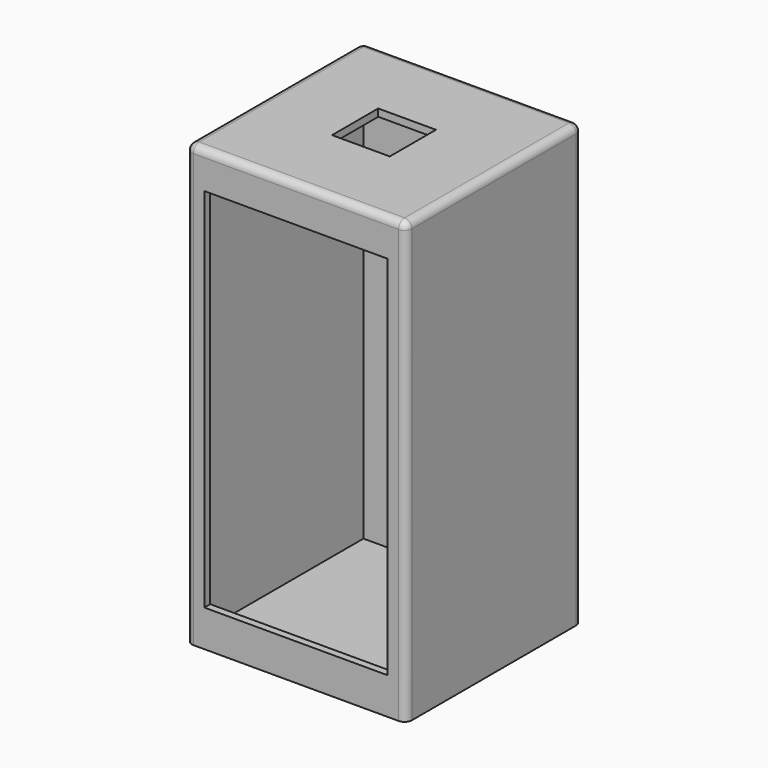
from build123d import *

# Parameters (mm, degrees)
F0_W     = 152.4
F0_H     = 304.8
F1_DEPTH = 76.2
F2_R     = 5.08
F3_T     = 5.08
F4_W     = 127
F4_H     = 254
F5_DEPTH = 25.4
F6_W     = 40
F6_H     = 40
F7_DEPTH = 5.08


# Not quite as in the source:
# - a shell that OpenCascade refuses in one call is made with other operations: the cavity is built on its own and cut out


with BuildPart() as f1:
    # F0 (on Front) → F1 (new body, symmetric)
    with BuildSketch(Plane.XZ):
        Rectangle(F0_W, F0_H)
    extrude(amount=F1_DEPTH, both=True)

    # F2
    f2_edges = [f1.edges().sort_by_distance(p)[0] for p in [
        (0, -76.2, 152.4),
        (76.2, 0, 152.4),
        (76.2, -76.2, 0),
        (76.2, 76.2, 0),
        (0, 76.2, 152.4),
        (-76.2, 0, 152.4),
        (-76.2, -76.2, 0),
        (-76.2, 76.2, 0),
    ]]
    fillet(f2_edges, radius=F2_R)

    # F3: shell of thickness 5.08, made by hand


with BuildPart() as f3_core1:
    # F3_t2: copy of F1
    add(f1.part)

    # the walls: a layer under each face that stays
    f3_faces = [f3_core1.faces().sort_by_distance(p)[0] for p in [
        (0, 0, -152.4),
        (0, 76.2, -2.54),
        (-76.2, 0, -2.54),
        (76.2, 0, -2.54),
        (0, -76.2, -2.54),
        (0, 0, 152.4),
    ]]
    thicken(f3_faces, amount=-F3_T, mode=Mode.SUBTRACT)


with BuildPart() as f1_1:
    add(f1.part)

    # what is left inside the walls is the cavity
    f3_cavity = [f3_core1.part.solids().sort_by_distance(p)[0] for p in [
        (-71.0692, 23.706667, 0),
    ]]
    add(f3_cavity, mode=Mode.SUBTRACT)

    # F4 (on face) → F5 (cut)
    with BuildSketch(Plane.XZ.offset(76.2)):
        Rectangle(F4_W, F4_H)
    extrude(amount=-F5_DEPTH, mode=Mode.SUBTRACT)

    # F6 (on face) → F7 (cut)
    with BuildSketch(Plane.XY.offset(152.4)):
        Rectangle(F6_W, F6_H)
    extrude(amount=-F7_DEPTH, mode=Mode.SUBTRACT)


solid = f1_1.part
